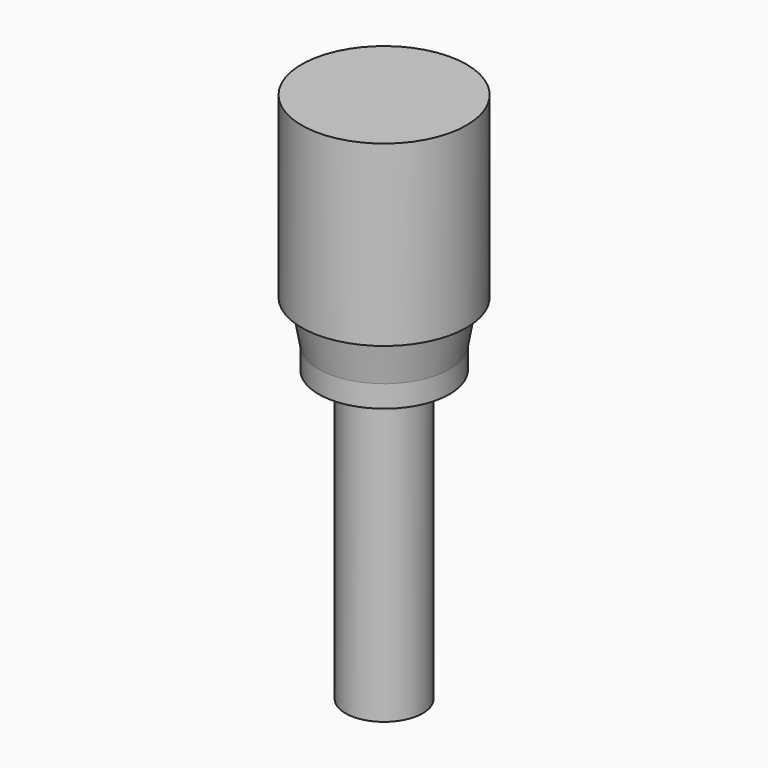
from build123d import *

# Parameters (mm, degrees)
F0_R      = 74.5643823595
F1_DEPTH  = 25
F1_FACE_R = 74.5643823595
F2_DEPTH  = 110
F2_TAPER  = -10
F3_R      = 57.2567690905
F2_FACE_R = 93.9603502375
F4_DEPTH  = 141
F5_R      = 44.0131368503
F6_DEPTH  = 330
F7_DEPTH  = 203


# Not quite as in the source:
# - a feature names something its author has since deleted; it is built from what else it names


with BuildPart() as f1:
    # F0 (on Top) → F1 (new body)
    with BuildSketch(Plane.XY):
        Circle(F0_R)
    extrude(amount=F1_DEPTH)

    # F1_face (on face) → F2 (join)
    with BuildSketch(Plane.XY.offset(25)):
        Circle(F1_FACE_R)
    extrude(amount=F2_DEPTH, taper=F2_TAPER)

    # F3 (on Top) + F2_face (on face) → F4 (join)
    with BuildSketch(Plane.XY):
        Circle(F3_R)
    with BuildSketch(Plane.XY.offset(135)):
        Circle(F2_FACE_R)
    extrude(amount=F4_DEPTH)

    # F5 (on Top) → F6 (join)
    with BuildSketch(Plane.XY):
        Circle(F5_R)
    extrude(amount=-F6_DEPTH)


with BuildPart() as f7:
    # F7 (new): a face of the model
    f7_faces = [f1.part.faces().sort_by_distance(p)[0] for p in [
        (0, 0, 276),
    ]]
    extrude(f7_faces, amount=-F7_DEPTH)


solid = Compound([f1.part, f7.part])
